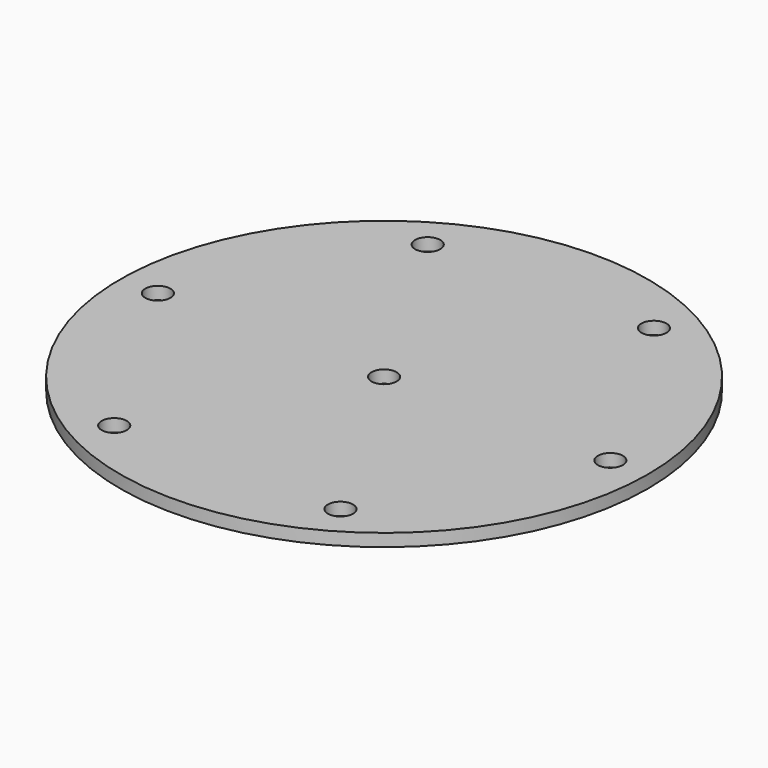
from build123d import *

# Parameters (mm, degrees)
F0_R     = 21
F1_DEPTH = 1
F2_D     = 2


# Not quite as in the source:
# - a feature names something its author has since deleted; it is built from what else it names


with BuildPart() as f1:
    # F0 (on Top) → F1 (new body)
    with BuildSketch(Plane.XY):
        Circle(F0_R)
    extrude(amount=F1_DEPTH)

    # F2 (through all)
    with Locations(Plane(origin=(0, 0, 0), x_dir=(1, 0, 0), z_dir=(0, 0, -1))):
        with Locations((-18, 0), (18, 0), (0, 0), (-9, 15.5884572681), (9, 15.5884572681), (9, -15.5884572681), (-9, -15.5884572681)):
            Hole(F2_D / 2)


solid = f1.part
